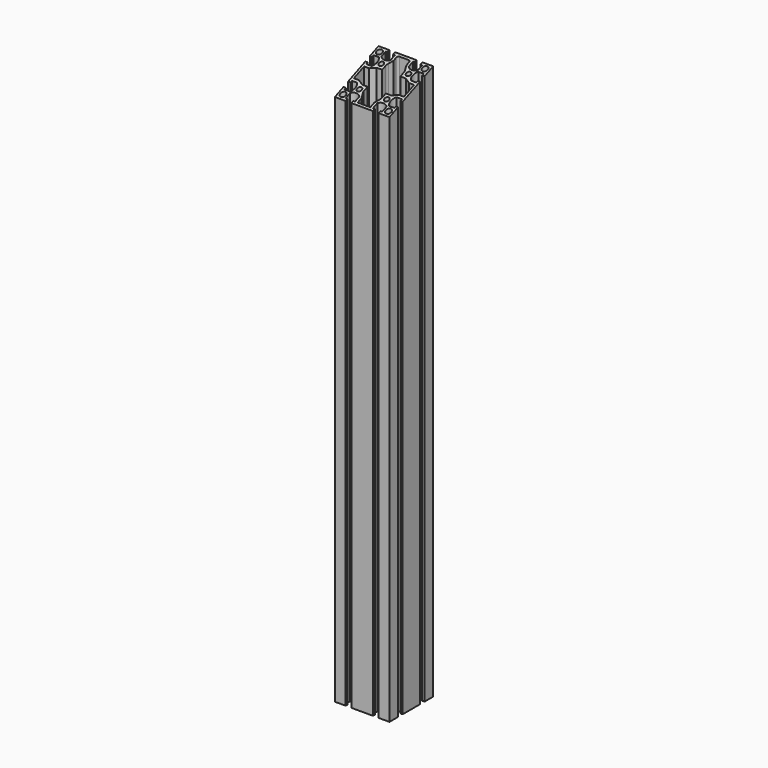
from build123d import *

# Parameters (mm, degrees)
F0_R          = 3
F0_R_2        = 2.5
F1_DEPTH      = 610
F2_R          = 2
F3_R          = 7
F5_DEPTH      = 30
F5_DEPTH_BACK = 30


# Not quite as in the source:
# - a feature names something its author has since deleted; it is built from what else it names


with BuildPart() as f1:
    # F0 (on Top) → F1 (new body)
    with BuildSketch(Plane.XY):
        with BuildLine():
            Line((18.15, -30), (30, -30))
            Line((30, -30), (30, -18.15))
            Line((30, -18.15), (27.5, -18.15))
            Line((27.5, -18.15), (27.5, -20.15))
            Line((27.5, -20.15), (21.5477069044, -20.15))
            ThreePointArc((21.5477069044, -20.15), (19.5, -15), (21.5477069044, -9.85))
            Line((21.5477069044, -9.85), (27.5, -9.85))
            Line((27.5, -9.85), (27.5, -11.85))
            Line((27.5, -11.85), (30, -11.85))
            Line((30, -11.85), (30, 11.85))
            Line((30, 11.85), (27.5, 11.85))
            Line((27.5, 11.85), (27.5, 9.85))
            Line((27.5, 9.85), (21.5477069044, 9.85))
            ThreePointArc((21.5477069044, 9.85), (19.5, 15), (21.5477069044, 20.15))
            Line((21.5477069044, 20.15), (27.5, 20.15))
            Line((27.5, 20.15), (27.5, 18.15))
            Line((27.5, 18.15), (30, 18.15))
            Line((30, 18.15), (30, 30))
            Line((30, 30), (18.15, 30))
            Line((18.15, 30), (18.15, 27.5))
            Line((18.15, 27.5), (20.15, 27.5))
            Line((20.15, 27.5), (20.15, 21.5477069044))
            ThreePointArc((20.15, 21.5477069044), (15, 19.5), (9.85, 21.5477069044))
            Line((9.85, 21.5477069044), (9.85, 27.5))
            Line((9.85, 27.5), (11.85, 27.5))
            Line((11.85, 27.5), (11.85, 30))
            Line((11.85, 30), (-11.85, 30))
            Line((-11.85, 30), (-11.85, 27.5))
            Line((-11.85, 27.5), (-9.85, 27.5))
            Line((-9.85, 27.5), (-9.85, 21.5477069044))
            ThreePointArc((-9.85, 21.5477069044), (-15, 19.5), (-20.15, 21.5477069044))
            Line((-20.15, 21.5477069044), (-20.15, 27.5))
            Line((-20.15, 27.5), (-18.15, 27.5))
            Line((-18.15, 27.5), (-18.15, 30))
            Line((-18.15, 30), (-30, 30))
            Line((-30, 30), (-30, 18.15))
            Line((-30, 18.15), (-27.5, 18.15))
            Line((-27.5, 18.15), (-27.5, 20.15))
            Line((-27.5, 20.15), (-21.5477069044, 20.15))
            ThreePointArc((-21.5477069044, 20.15), (-19.5, 15), (-21.5477069044, 9.85))
            Line((-21.5477069044, 9.85), (-27.5, 9.85))
            Line((-27.5, 9.85), (-27.5, 11.85))
            Line((-27.5, 11.85), (-30, 11.85))
            Line((-30, 11.85), (-30, -11.85))
            Line((-30, -11.85), (-27.5, -11.85))
            Line((-27.5, -11.85), (-27.5, -9.85))
            Line((-27.5, -9.85), (-21.5477069044, -9.85))
            ThreePointArc((-21.5477069044, -9.85), (-19.5, -15), (-21.5477069044, -20.15))
            Line((-21.5477069044, -20.15), (-27.5, -20.15))
            Line((-27.5, -20.15), (-27.5, -18.15))
            Line((-27.5, -18.15), (-30, -18.15))
            Line((-30, -18.15), (-30, -30))
            Line((-30, -30), (-18.15, -30))
            Line((-18.15, -30), (-18.15, -27.5))
            Line((-18.15, -27.5), (-20.15, -27.5))
            Line((-20.15, -27.5), (-20.15, -21.5477069044))
            ThreePointArc((-20.15, -21.5477069044), (-15, -19.5), (-9.85, -21.5477069044))
            Line((-9.85, -21.5477069044), (-9.85, -27.5))
            Line((-9.85, -27.5), (-11.85, -27.5))
            Line((-11.85, -27.5), (-11.85, -30))
            Line((-11.85, -30), (11.85, -30))
            Line((11.85, -30), (11.85, -27.5))
            Line((11.85, -27.5), (9.85, -27.5))
            Line((9.85, -27.5), (9.85, -21.5477069044))
            ThreePointArc((9.85, -21.5477069044), (15, -19.5), (20.15, -21.5477069044))
            Line((20.15, -21.5477069044), (20.15, -27.5))
            Line((20.15, -27.5), (18.15, -27.5))
            Line((18.15, -27.5), (18.15, -30))
        make_face()
        with Locations((-25, -25)):
            Circle(F0_R, mode=Mode.SUBTRACT)
        with Locations((-15, -15)):
            Circle(F0_R_2, mode=Mode.SUBTRACT)
        with Locations((25, -25)):
            Circle(F0_R, mode=Mode.SUBTRACT)
        with Locations((15, -15)):
            Circle(F0_R_2, mode=Mode.SUBTRACT)
        with Locations((-25, 25)):
            Circle(F0_R, mode=Mode.SUBTRACT)
        with Locations((-15, 15)):
            Circle(F0_R_2, mode=Mode.SUBTRACT)
        Polygon((-7, 22), (-7, 27.5), (0, 27.5), (7, 27.5), (7, 22), (10, 16), (10, 10), (16, 10), (22, 7), (27.5, 7), (27.5, 0), (27.5, -7), (22, -7), (16, -10), (10, -10), (10, -16), (7, -22), (7, -27.5), (0, -27.5), (-7, -27.5), (-7, -22), (-10, -16), (-10, -10), (-16, -10), (-22, -7), (-27.5, -7), (-27.5, 0), (-27.5, 7), (-22, 7), (-16, 10), (-10, 10), (-10, 16), align=None, mode=Mode.SUBTRACT)
        with Locations((15, 15)):
            Circle(F0_R_2, mode=Mode.SUBTRACT)
        with Locations((25, 25)):
            Circle(F0_R, mode=Mode.SUBTRACT)
    extrude(amount=F1_DEPTH)

    # F2
    f2_edges = [f1.edges().sort_by_distance(p)[0] for p in [
        (-7, 27.5, 305),
        (7, 27.5, 305),
    ]]
    fillet(f2_edges, radius=F2_R)

    # F3
    f3_edges = [f1.edges().sort_by_distance(p)[0] for p in [
        (-10, 16, 305),
        (10, 16, 305),
    ]]
    fillet(f3_edges, radius=F3_R)

    # F4 (on Right) → F5 (cut, two sides)
    with BuildSketch(Plane.YZ) as f5_sk:
        Polygon((-66.9285170742, 844.0061405012), (-249.6042822322, 768.3393610558), (-152.6757651581, 534.3332205546), (30, 610), align=None)
    extrude(amount=F5_DEPTH, mode=Mode.SUBTRACT)
    extrude(f5_sk.sketch, amount=-F5_DEPTH_BACK, mode=Mode.SUBTRACT)


solid = f1.part
